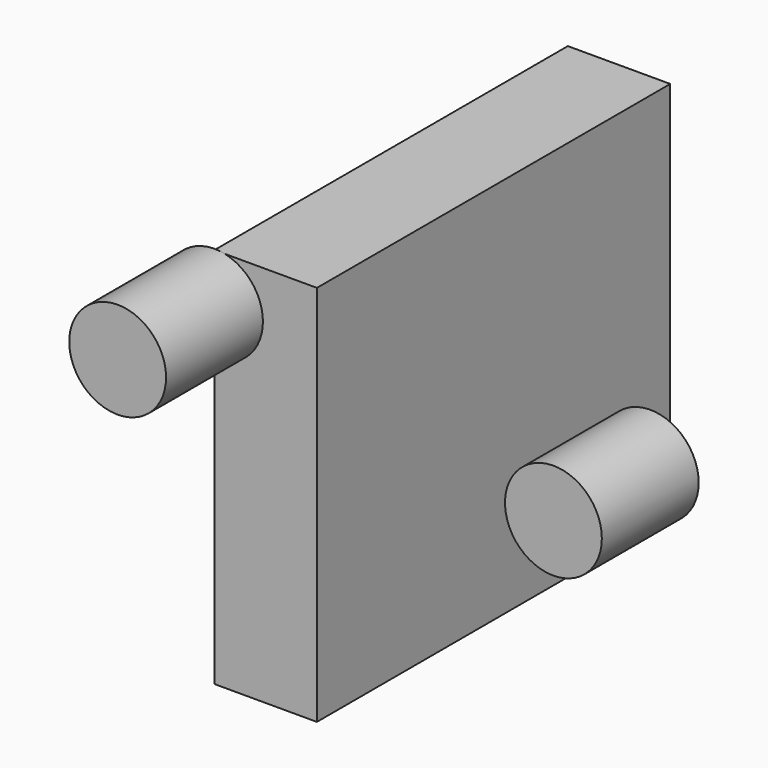
from build123d import *

# Parameters (mm, degrees)
F0_R     = 10
F1_DEPTH = 25
F2_W     = 21.1537368596
F2_H     = 78.9189003408
F3_DEPTH = 91.2176873535


# Not quite as in the source:
# - a feature names something its author has since deleted; it is built from what else it names


with BuildPart() as f1:
    # F0 (on Front) → F1 (new body)
    with BuildSketch(Plane.XZ):
        Circle(F0_R)
    extrude(amount=F1_DEPTH)

    # F2 (on face) → F3 (join)
    with BuildSketch(Plane.XZ):
        with Locations((10.5768684298, -29.6896714717)):
            Rectangle(F2_W, F2_H)
    extrude(amount=-F3_DEPTH)


with BuildPart() as f1b:
    # F0 (on Front) → F1, piece 2 (new body)
    with BuildSketch(Plane.XZ):
        with Locations((90, 0)):
            Circle(F0_R)
    extrude(amount=F1_DEPTH)


solid = Compound([f1.part, f1b.part])
